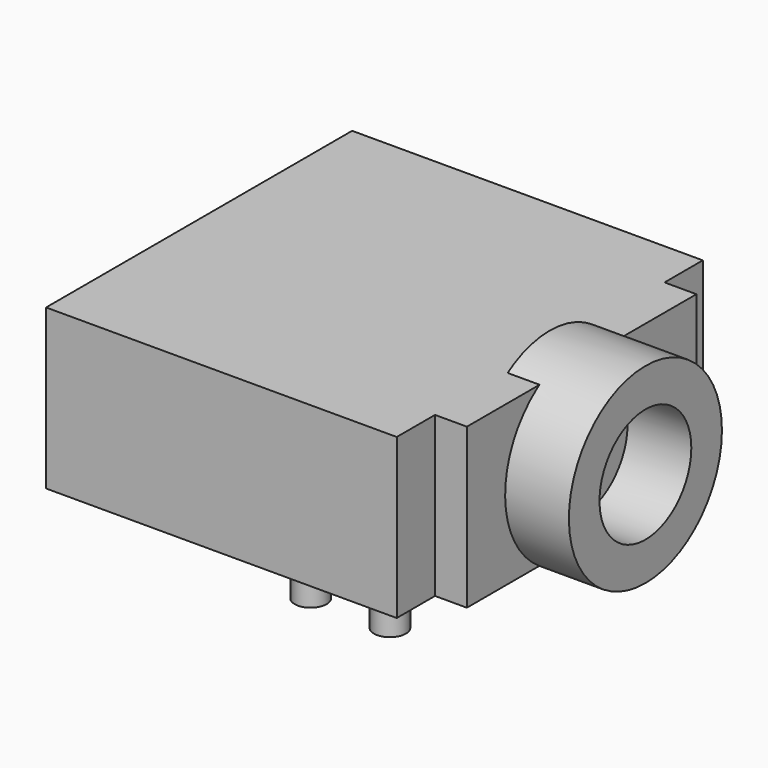
from build123d import *

# Parameters (mm, degrees)
F0_R     = 1.8
F1_DEPTH = 3
F2_W     = 9
F2_H     = 5
F3_DEPTH = 1
F4_W     = 12
F4_H     = 5
F5_DEPTH = 11
F6_R     = 0.5
F7_DEPTH = 1


# Not quite as in the source:
# - a feature names something its author has since deleted; it is built from what else it names


with BuildPart() as f1:
    # F0 (on Right) → F1 (new body)
    with BuildSketch(Plane.YZ):
        with BuildLine():
            ThreePointArc((1.6524272508, -2.5038938038), (2.6417117322, -1.421745098), (3, 0))
            ThreePointArc((3, 0), (-1.421745098, 2.6417117322), (-1.6524272508, -2.5038938038))
            Line((-1.6524272508, -2.5038938038), (1.6524272508, -2.5038938038))
        make_face()
        Circle(F0_R, mode=Mode.SUBTRACT)
        with BuildLine():
            Line((1.6524272508, -2.5038938038), (-1.6524272508, -2.5038938038))
            ThreePointArc((-1.6524272508, -2.5038938038), (0, -3), (1.6524272508, -2.5038938038))
        make_face()
    extrude(amount=-F1_DEPTH)


with BuildPart() as f3:
    # F2 (on face) → F3 (new body)
    with BuildSketch(Plane(origin=(-3, 0, 0), x_dir=(0, -1, 0), z_dir=(-1, 0, 0))):
        Rectangle(F2_W, F2_H)
    extrude(amount=-F3_DEPTH)

    # F4 (on face) → F5 (join)
    with BuildSketch(Plane(origin=(-3, 0, 0), x_dir=(0, -1, 0), z_dir=(-1, 0, 0))):
        Rectangle(F4_W, F4_H)
    extrude(amount=F5_DEPTH)


with BuildPart() as f7:
    # F6 (on face) → F7 (new body)
    with BuildSketch(Plane(origin=(0, 0, -2.5), x_dir=(1, 0, 0), z_dir=(0, 0, -1))):
        with Locations((-4.0077906769, 5.0080687183)):
            Circle(F6_R)
    extrude(amount=F7_DEPTH)


with BuildPart() as f7b:
    # F6 (on face) → F7, piece 2 (new body)
    with BuildSketch(Plane(origin=(0, 0, -2.5), x_dir=(1, 0, 0), z_dir=(0, 0, -1))):
        with Locations((-11.5011356074, 0)):
            Circle(F6_R)
    extrude(amount=F7_DEPTH)


with BuildPart() as f7c:
    # F6 (on face) → F7, piece 3 (new body)
    with BuildSketch(Plane(origin=(0, 0, -2.5), x_dir=(1, 0, 0), z_dir=(0, 0, -1))):
        with Locations((-6.5, -5)):
            Circle(F6_R)
    extrude(amount=F7_DEPTH)


with BuildPart() as f7d:
    # F6 (on face) → F7, piece 4 (new body)
    with BuildSketch(Plane(origin=(0, 0, -2.5), x_dir=(1, 0, 0), z_dir=(0, 0, -1))):
        with Locations((-6.5, 5)):
            Circle(F6_R)
    extrude(amount=F7_DEPTH)


with BuildPart() as f7e:
    # F6 (on face) → F7, piece 5 (new body)
    with BuildSketch(Plane(origin=(0, 0, -2.5), x_dir=(1, 0, 0), z_dir=(0, 0, -1))):
        with Locations((-4.0077906769, -5.0080687183)):
            Circle(F6_R)
    extrude(amount=F7_DEPTH)


solid = Compound([f1.part, f3.part, f7.part, f7b.part, f7c.part, f7d.part, f7e.part])
